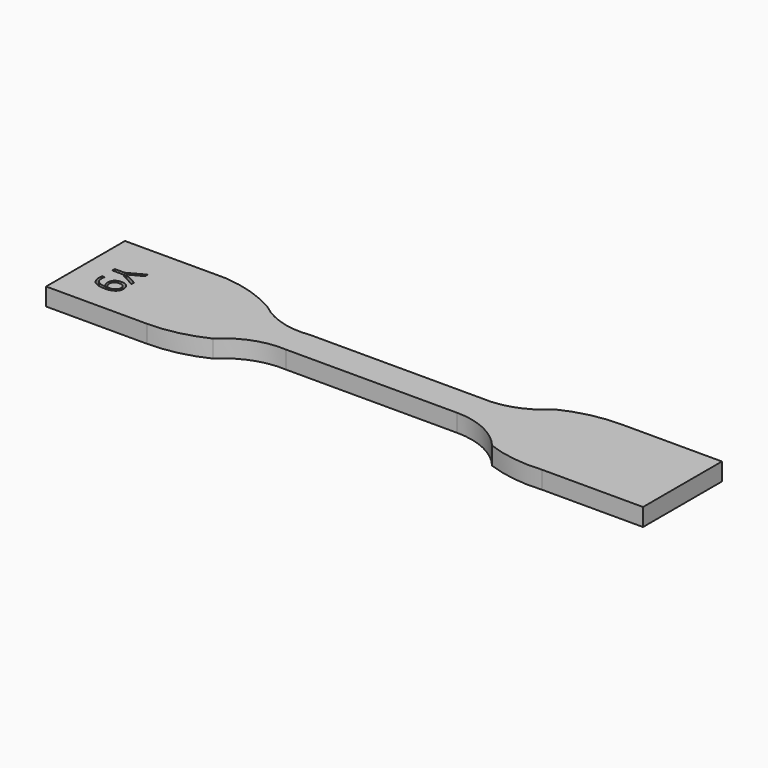
from build123d import *

# Parameters (mm, degrees)
F1_DEPTH     = 3.4
F2_TEXT_SIZE = 7.0564552314
F3_DEPTH     = 1


# Not quite as in the source:
# - Text() gives the source's letters only with a copy of the font that has no kerning and outlines rounded to 1/6400 em; it was checked with that copy


with BuildPart() as f1:
    # F0 (on Top) → F1 (new body)
    with BuildSketch(Plane.XY):
        with BuildLine():
            Line((-14.4320548165, 19.7811394548), (-33.8720548165, 19.7811394548))
            Line((-33.8720548165, 19.7811394548), (-33.8720548165, 0.7811394548))
            Line((-33.8720548165, 0.7811394548), (-14.4320548165, 0.7811394548))
            ThreePointArc((-14.4320548165, 0.7811394548), (-8.9053122052, 1.3996892086), (-3.6520548165, 3.2247301661))
            ThreePointArc((-3.6520548165, 3.2247301661), (1.3014698263, 6.4128780055), (7.1279451835, 7.2811394548))
            Line((7.1279451835, 7.2811394548), (40.1279451835, 7.2811394548))
            ThreePointArc((40.1279451835, 7.2811394548), (46.0837574042, 5.9511158081), (50.9079451835, 2.2137538538))
            ThreePointArc((50.9079451835, 2.2137538538), (56.2191047011, 0.9041953221), (61.6879451835, 0.7811394548))
            Line((61.6879451835, 0.7811394548), (81.1279451835, 0.7811394548))
            Line((81.1279451835, 0.7811394548), (81.1279451835, 19.7811394548))
            Line((81.1279451835, 19.7811394548), (61.6879451835, 19.7811394548))
            ThreePointArc((61.6879451835, 19.7811394548), (56.1612025723, 19.162589701), (50.9079451835, 17.3375487435))
            ThreePointArc((50.9079451835, 17.3375487435), (45.9544205407, 14.1494009041), (40.1279451835, 13.2811394548))
            Line((40.1279451835, 13.2811394548), (7.1279451835, 13.2811394548))
            ThreePointArc((7.1279451835, 13.2811394548), (1.4167452884, 13.6925537245), (-3.6520548165, 16.3560723447))
            ThreePointArc((-3.6520548165, 16.3560723447), (-8.8458057958, 18.686276846), (-14.4320548165, 19.7811394548))
        make_face()
    extrude(amount=F1_DEPTH)

    # F2 (on face) → F3 (cut)
    with BuildSketch(Plane.XY.offset(3.4)):
        with Locations(Location((-29.3720550835, 13.353464842), (0, 0, -90))):
            Text('Y9', F2_TEXT_SIZE, font='Open Sans', text_align=(TextAlign.LEFT, TextAlign.BOTTOM))
    extrude(amount=-F3_DEPTH, mode=Mode.SUBTRACT)


solid = f1.part
